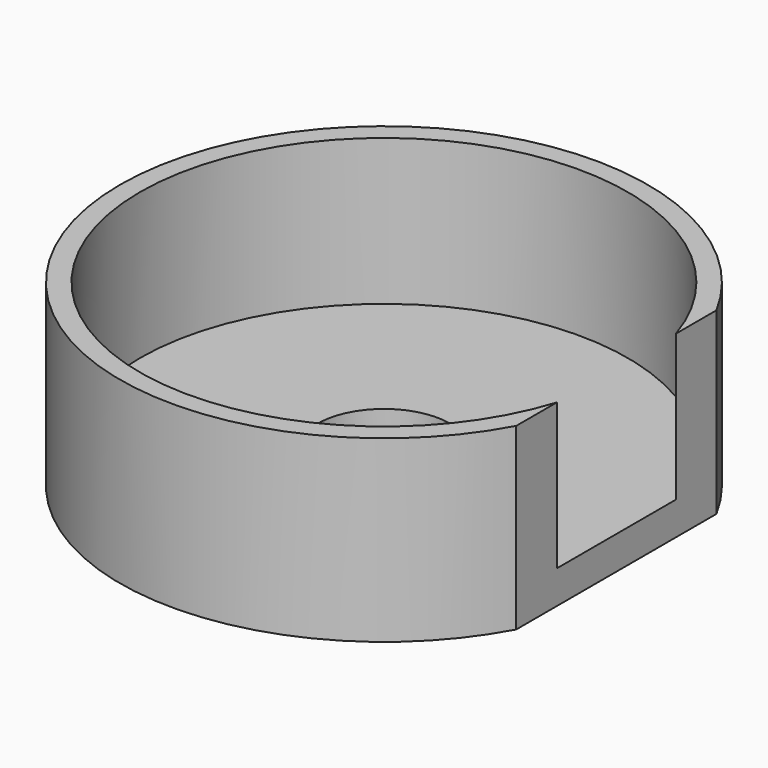
from build123d import *

# Parameters (mm, degrees)
F0_R     = 15.9
F0_R_2   = 4
F1_DEPTH = 10
F2_T     = -1.2
F3_DEPTH = 10.001
F4_DEPTH = 0.8
F5_W     = 2
F5_H     = 3.5
F6_DEPTH = 10.801


# Not quite as in the source:
# - a feature names something its author has since deleted; it is built from what else it names


with BuildPart() as f1:
    # F0 (on Top) → F1 (new body)
    with BuildSketch(Plane.XY):
        Circle(F0_R)
        Circle(F0_R_2, mode=Mode.SUBTRACT)
        Circle(F0_R_2)
    extrude(amount=F1_DEPTH)

    # F2
    f2_openings = [f1.faces().sort_by_distance(p)[0] for p in [
        (0, 0, 10),
    ]]
    offset(amount=F2_T, openings=f2_openings)

    # F0 (on Top) → F3 (cut, through all)
    with BuildSketch(Plane.XY):
        Circle(F0_R_2)
    extrude(amount=F3_DEPTH, mode=Mode.SUBTRACT)

    # F0 (on Top) → F4 (join)
    with BuildSketch(Plane.XY):
        Circle(F0_R)
        Circle(F0_R_2, mode=Mode.SUBTRACT)
    extrude(amount=-F4_DEPTH)

    # F5 (on face) → F6 (cut, through all)
    with BuildSketch(Plane(origin=(0, 0, -0.8), x_dir=(1, 0, 0), z_dir=(0, 0, -1))):
        with Locations((5.9, 0)):
            Rectangle(F5_W, F5_H)
        with BuildLine():
            ThreePointArc((15.9, 0), (15.4176846511, 3.8865151486), (14, 7.5372408745))
            Line((14, 7.5372408745), (14, -7.5372408745))
            ThreePointArc((14, -7.5372408745), (15.4176846511, -3.8865151486), (15.9, 0))
        make_face()
    extrude(amount=-F6_DEPTH, mode=Mode.SUBTRACT)


solid = f1.part
